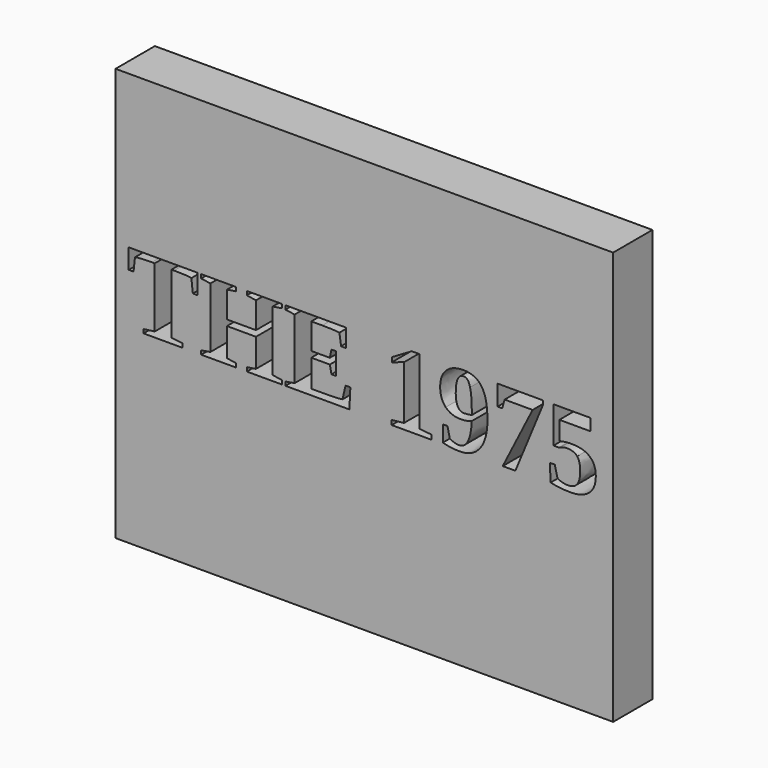
from build123d import *

# Parameters (mm, degrees)
F0_W     = 128.5621747375
F0_H     = 106.7495681345
F1_DEPTH = 12.7


with BuildPart() as f1:
    # F0 (on Front) → F1 (new body)
    with BuildSketch(Plane.XZ):
        with Locations((1.2247897685, -6.9555658847)):
            Rectangle(F0_W, F0_H)
        with BuildLine():
            Line((-45.696739094, -11.4172368776), (-55.8424323255, -11.4172368776))
            Line((-55.8424323255, -11.4172368776), (-55.8424323255, -10.4197301692))
            Line((-55.8424323255, -10.4197301692), (-52.9330377593, -10.0478526683))
            Line((-52.9330377593, -10.0478526683), (-52.9330377593, 5.466001665))
            Line((-52.9330377593, 5.466001665), (-53.6286674376, 5.466001665))
            add(Edge.make_bspline(
                [(-53.6286674376, 5.466001665), (-56.7611885043, 5.466001665), (-58.0299470369, 5.1947498407)],
                knots=[0, 0, 0, 1, 1, 1], degree=2))
            Line((-58.0299470369, 5.1947498407), (-58.4018245378, 1.7909769498))
            Line((-58.4018245378, 1.7909769498), (-59.6443328939, 1.7909769498))
            Line((-59.6443328939, 1.7909769498), (-59.6443328939, 6.9185114333))
            Line((-59.6443328939, 6.9185114333), (-41.8292130843, 6.9185114333))
            Line((-41.8292130843, 6.9185114333), (-41.8292130843, 1.7909769498))
            Line((-41.8292130843, 1.7909769498), (-43.089221558, 1.7909769498))
            Line((-43.089221558, 1.7909769498), (-43.4567240296, 5.1947498407))
            add(Edge.make_bspline(
                [(-43.4567240296, 5.1947498407), (-44.5898566501, 5.4397514884), (-47.9411291879, 5.4397514884)],
                knots=[0, 0, 0, 1, 1, 1], degree=2))
            Line((-47.9411291879, 5.4397514884), (-48.6105086896, 5.4397514884))
            Line((-48.6105086896, 5.4397514884), (-48.6105086896, -10.0478526683))
            Line((-48.6105086896, -10.0478526683), (-45.696739094, -10.4197301692))
            Line((-45.696739094, -10.4197301692), (-45.696739094, -11.4172368776))
        make_face(mode=Mode.SUBTRACT)
        Polygon((-31.9153964122, -11.4172368776), (-40.9279570232, -11.4172368776), (-40.9279570232, -10.4066050809), (-38.5741911937, -10.0478526683), (-38.5741911937, 5.549127224), (-40.9279570232, 5.9210047249), (-40.9279570232, 6.9185114333), (-31.9153964122, 6.9185114333), (-31.9153964122, 5.9210047249), (-34.2691622417, 5.549127224), (-34.2691622417, -1.2321683813), (-26.7747368405, -1.2321683813), (-26.7747368405, 5.549127224), (-29.1285026699, 5.9210047249), (-29.1285026699, 6.9185114333), (-20.0896918824, 6.9185114333), (-20.0896918824, 5.9210047249), (-22.4565828002, 5.549127224), (-22.4565828002, -10.0478526683), (-20.0896918824, -10.4066050809), (-20.0896918824, -11.4172368776), (-29.1285026699, -11.4172368776), (-29.1285026699, -10.4066050809), (-26.7747368405, -10.0478526683), (-26.7747368405, -2.7371785028), (-34.2691622417, -2.7371785028), (-34.2691622417, -10.0478526683), (-31.9153964122, -10.4066050809), align=None, mode=Mode.SUBTRACT)
        with BuildLine():
            Line((-19.1490605565, -11.4172368776), (-19.1490605565, -10.4197301692))
            Line((-19.1490605565, -10.4197301692), (-16.7952947271, -10.0478526683))
            Line((-16.7952947271, -10.0478526683), (-16.7952947271, 5.5622523123))
            Line((-16.7952947271, 5.5622523123), (-19.1490605565, 5.9210047249))
            Line((-19.1490605565, 5.9210047249), (-19.1490605565, 6.9185114333))
            Line((-19.1490605565, 6.9185114333), (-3.5345805466, 6.9185114333))
            Line((-3.5345805466, 6.9185114333), (-3.5345805466, 2.2547300686))
            Line((-3.5345805466, 2.2547300686), (-4.7770889027, 2.2547300686))
            Line((-4.7770889027, 2.2547300686), (-5.2145918449, 5.2210000173))
            add(Edge.make_bspline(
                [(-5.2145918449, 5.2210000173), (-6.7458521429, 5.4135013119), (-9.6464966502, 5.4135013119)],
                knots=[0, 0, 0, 1, 1, 1], degree=2))
            Line((-9.6464966502, 5.4135013119), (-12.490265775, 5.4135013119))
            Line((-12.490265775, 5.4135013119), (-12.490265775, -1.3152939404))
            Line((-12.490265775, -1.3152939404), (-7.6908584982, -1.3152939404))
            Line((-7.6908584982, -1.3152939404), (-7.2664806442, 0.7103446824))
            Line((-7.2664806442, 0.7103446824), (-6.0502224647, 0.7103446824))
            Line((-6.0502224647, 0.7103446824), (-6.0502224647, -4.9246932142))
            Line((-6.0502224647, -4.9246932142), (-7.2664806442, -4.9246932142))
            Line((-7.2664806442, -4.9246932142), (-7.6908584982, -2.8465542384))
            Line((-7.6908584982, -2.8465542384), (-12.490265775, -2.8465542384))
            Line((-12.490265775, -2.8465542384), (-12.490265775, -9.9122267562))
            Line((-12.490265775, -9.9122267562), (-9.0296175016, -9.9122267562))
            add(Edge.make_bspline(
                [(-9.0296175016, -9.9122267562), (-5.5033437868, -9.9122267562), (-4.4095864311, -9.693475285)],
                knots=[0, 0, 0, 1, 1, 1], degree=2))
            Line((-4.4095864311, -9.693475285), (-3.6308311939, -6.3028274824))
            Line((-3.6308311939, -6.3028274824), (-2.3839478084, -6.3028274824))
            Line((-2.3839478084, -6.3028274824), (-2.6464495738, -11.4172368776))
            Line((-2.6464495738, -11.4172368776), (-19.1490605565, -11.4172368776))
        make_face(mode=Mode.SUBTRACT)
        Polygon((15.418046913, 7.0672624337), (15.418046913, -9.9122267562), (18.6030683327, -10.2403539629), (18.6030683327, -11.4172368776), (8.2954990126, -11.4172368776), (8.2954990126, -10.2403539629), (11.4673953442, -9.9122267562), (11.4673953442, 3.9084911904), (8.3086241009, 2.8716092172), (8.3086241009, 4.0309920143), (13.4755338492, 7.0672624337), align=None, mode=Mode.SUBTRACT)
        with BuildLine():
            add(Edge.make_bspline(
                [(22.2452803272, -2.8181165471), (20.8168332207, -1.3415441169), (20.8168332207, 1.327223831)],
                knots=[0, 0, 0, 1, 1, 1], degree=2))
            add(Edge.make_bspline(
                [(20.8168332207, 1.327223831), (20.8168332207, 4.1141175733), (22.4159064747, 5.6191276947)],
                knots=[0, 0, 0, 1, 1, 1], degree=2))
            add(Edge.make_bspline(
                [(22.4159064747, 5.6191276947), (24.0149797287, 7.1241378162), (26.8587488536, 7.1241378162)],
                knots=[0, 0, 0, 1, 1, 1], degree=2))
            add(Edge.make_bspline(
                [(26.8587488536, 7.1241378162), (30.0743954793, 7.1241378162), (31.5575304536, 4.866622634)],
                knots=[0, 0, 0, 1, 1, 1], degree=2))
            add(Edge.make_bspline(
                [(31.5575304536, 4.866622634), (33.040665428, 2.6091074519), (33.040665428, -2.2034249132)],
                knots=[0, 0, 0, 1, 1, 1], degree=2))
            add(Edge.make_bspline(
                [(33.040665428, -2.2034249132), (33.040665428, -5.2921956857), (32.1722220875, -7.411897441)],
                knots=[0, 0, 0, 1, 1, 1], degree=2))
            add(Edge.make_bspline(
                [(32.1722220875, -7.411897441), (31.3037787471, -9.5315991964), (29.6762678018, -10.6122314638)],
                knots=[0, 0, 0, 1, 1, 1], degree=2))
            add(Edge.make_bspline(
                [(29.6762678018, -10.6122314638), (28.0487568566, -11.6928637312), (25.7649914979, -11.6928637312)],
                knots=[0, 0, 0, 1, 1, 1], degree=2))
            add(Edge.make_bspline(
                [(25.7649914979, -11.6928637312), (23.4987262569, -11.6928637312), (21.5124628989, -11.1022347592)],
                knots=[0, 0, 0, 1, 1, 1], degree=2))
            Line((21.5124628989, -11.1022347592), (21.5124628989, -6.9328317192))
            Line((21.5124628989, -6.9328317192), (22.7024709019, -6.9328317192))
            Line((22.7024709019, -6.9328317192), (23.293099874, -9.5840995495))
            add(Edge.make_bspline(
                [(23.293099874, -9.5840995495), (23.7699780811, -9.9253518444), (24.4327950386, -10.117853139)],
                knots=[0, 0, 0, 1, 1, 1], degree=2))
            add(Edge.make_bspline(
                [(24.4327950386, -10.117853139), (25.0956119962, -10.3103544336), (25.7124911448, -10.3103544336)],
                knots=[0, 0, 0, 1, 1, 1], degree=2))
            add(Edge.make_bspline(
                [(25.7124911448, -10.3103544336), (27.1868760603, -10.3103544336), (28.0137566212, -8.6347181647)],
                knots=[0, 0, 0, 1, 1, 1], degree=2))
            add(Edge.make_bspline(
                [(28.0137566212, -8.6347181647), (28.8406371821, -6.9590818958), (28.9806381236, -3.7871855643)],
                knots=[0, 0, 0, 1, 1, 1], degree=2))
            add(Edge.make_bspline(
                [(28.9806381236, -3.7871855643), (27.5587535612, -4.2946889773), (26.1499940871, -4.2946889773)],
                knots=[0, 0, 0, 1, 1, 1], degree=2))
            add(Edge.make_bspline(
                [(26.1499940871, -4.2946889773), (23.6737274338, -4.2946889773), (22.2452803272, -2.8181165471)],
                knots=[0, 0, 0, 1, 1, 1], degree=2))
        make_face(mode=Mode.SUBTRACT)
        Polygon((37.4681952038, 3.8691159256), (36.8425659964, 1.6816012142), (35.6525579934, 1.6816012142), (35.6525579934, 6.9185114333), (47.3688867876, 6.9185114333), (47.3688867876, 5.8378791659), (40.2463388873, -11.4172368776), (36.9781919085, -11.4172368776), (44.7001188397, 3.8691159256), align=None, mode=Mode.SUBTRACT)
        with BuildLine():
            add(Edge.make_bspline(
                [(51.6082902983, -0.9434164394), (53.2751765084, -0.5759139679), (54.6139355118, -0.5759139679)],
                knots=[0, 0, 0, 1, 1, 1], degree=2))
            add(Edge.make_bspline(
                [(54.6139355118, -0.5759139679), (57.8689574023, -0.5759139679), (59.4483430239, -1.9146729713)],
                knots=[0, 0, 0, 1, 1, 1], degree=2))
            add(Edge.make_bspline(
                [(59.4483430239, -1.9146729713), (61.0277286456, -3.2534319747), (61.0277286456, -5.9615751874)],
                knots=[0, 0, 0, 1, 1, 1], degree=2))
            add(Edge.make_bspline(
                [(61.0277286456, -5.9615751874), (61.0277286456, -8.7222187532), (59.3105295971, -10.2075412422)],
                knots=[0, 0, 0, 1, 1, 1], degree=2))
            add(Edge.make_bspline(
                [(59.3105295971, -10.2075412422), (57.5933305487, -11.6928637312), (54.3951840406, -11.6928637312)],
                knots=[0, 0, 0, 1, 1, 1], degree=2))
            add(Edge.make_bspline(
                [(54.3951840406, -11.6928637312), (51.853291946, -11.6928637312), (49.3376500279, -11.141610024)],
                knots=[0, 0, 0, 1, 1, 1], degree=2))
            Line((49.3376500279, -11.141610024), (49.1713989098, -6.7009551598))
            Line((49.1713989098, -6.7009551598), (50.4314073836, -6.7009551598))
            Line((50.4314073836, -6.7009551598), (51.1401621501, -9.640974932))
            add(Edge.make_bspline(
                [(51.1401621501, -9.640974932), (51.6739157396, -9.9384769327), (52.4526709769, -10.1244156832)],
                knots=[0, 0, 0, 1, 1, 1], degree=2))
            add(Edge.make_bspline(
                [(52.4526709769, -10.1244156832), (53.2314262141, -10.3103544336), (53.861430451, -10.3103544336)],
                knots=[0, 0, 0, 1, 1, 1], degree=2))
            add(Edge.make_bspline(
                [(53.861430451, -10.3103544336), (57.007076606, -10.3103544336), (57.007076606, -6.0972010995)],
                knots=[0, 0, 0, 1, 1, 1], degree=2))
            add(Edge.make_bspline(
                [(57.007076606, -6.0972010995), (57.007076606, -3.9096863881), (56.2064462216, -2.9318673121)],
                knots=[0, 0, 0, 1, 1, 1], degree=2))
            add(Edge.make_bspline(
                [(56.2064462216, -2.9318673121), (55.4058158373, -1.9540482361), (53.6558040682, -1.9540482361)],
                knots=[0, 0, 0, 1, 1, 1], degree=2))
            add(Edge.make_bspline(
                [(53.6558040682, -1.9540482361), (52.6845475363, -1.9540482361), (51.8795421225, -2.3128006488)],
                knots=[0, 0, 0, 1, 1, 1], degree=2))
            Line((51.8795421225, -2.3128006488), (51.4551642685, -2.4878018257))
            Line((51.4551642685, -2.4878018257), (50.0901550886, -2.4878018257))
            Line((50.0901550886, -2.4878018257), (50.0901550886, 6.9185114333))
            Line((50.0901550886, 6.9185114333), (59.6583444362, 6.9185114333))
            Line((59.6583444362, 6.9185114333), (59.6583444362, 3.8691159256))
            Line((59.6583444362, 3.8691159256), (51.6082902983, 3.8691159256))
            Line((51.6082902983, 3.8691159256), (51.6082902983, -0.9434164394))
        make_face(mode=Mode.SUBTRACT)
    extrude(amount=F1_DEPTH)


with BuildPart() as f1b:
    # F0 (on Front) → F1, piece 2 (new body)
    with BuildSketch(Plane.XZ):
        with BuildLine():
            add(Edge.make_bspline(
                [(26.8893740595, 5.7416285186), (24.8374852602, 5.7416285186), (24.8374852602, 1.2703484485)],
                knots=[0, 0, 0, 1, 1, 1], degree=2))
            add(Edge.make_bspline(
                [(24.8374852602, 1.2703484485), (24.8374852602, -2.6409278555), (26.9681245891, -2.6409278555)],
                knots=[0, 0, 0, 1, 1, 1], degree=2))
            add(Edge.make_bspline(
                [(26.9681245891, -2.6409278555), (28.0093815918, -2.6409278555), (29.0200133884, -2.3915511784)],
                knots=[0, 0, 0, 1, 1, 1], degree=2))
            Line((29.0200133884, -2.3915511784), (29.0200133884, -2.2034249132))
            add(Edge.make_bspline(
                [(29.0200133884, -2.2034249132), (29.0200133884, 1.7472266556), (28.5475102108, 3.7444275871)],
                knots=[0, 0, 0, 1, 1, 1], degree=2))
            add(Edge.make_bspline(
                [(28.5475102108, 3.7444275871), (28.0750070331, 5.7416285186), (26.8893740595, 5.7416285186)],
                knots=[0, 0, 0, 1, 1, 1], degree=2))
        make_face()
    extrude(amount=F1_DEPTH)


solid = Compound([f1.part, f1b.part])
